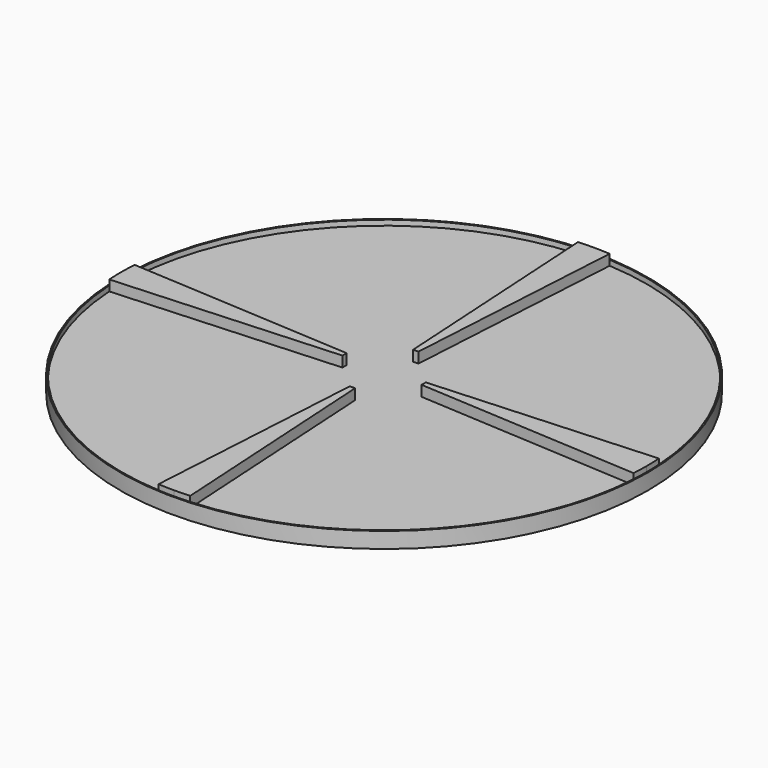
from build123d import *

# Parameters (mm, degrees)
F0_W      = 150
F0_H      = 140
F1_DEPTH  = 2
F2_R      = 2.5
F3_DEPTH  = 2.001
F4_R      = 50
F4_R_2    = 49.75
F5_DEPTH  = 1
F7_DEPTH  = 2
F8_DEPTH  = 25
F9_DEPTH  = 2.001
F10_DEPTH = 25


# Not quite as in the source:
# - a feature names something its author has since deleted; it is built from what else it names


with BuildPart() as f1:
    # F0 (on Top) → F1 (new body)
    with BuildSketch(Plane.XY):
        Rectangle(F0_W, F0_H)
    extrude(amount=F1_DEPTH)

    # F2 (on face) → F3 (cut, through all)
    with BuildSketch(Plane.XY.offset(2)):
        Polygon((-75, 70), (-75, 41.5), (-46.5, 70), align=None)
        with Locations((-64, 57.6)):
            Circle(F2_R, mode=Mode.SUBTRACT)
        Polygon((-46.5, -70), (-75, -41.5), (-75, -70), align=None)
        with Locations((-64, -57.6)):
            Circle(F2_R, mode=Mode.SUBTRACT)
        with BuildLine():
            Line((-67.1845650673, -7), (-67.1845650673, 7))
            ThreePointArc((-67.1845650673, 7), (-67.9167981143, 8.767766953), (-69.6845650673, 9.5))
            Line((-69.6845650673, 9.5), (-75, 9.5))
            Line((-75, 9.5), (-75, -9.5))
            Line((-75, -9.5), (-69.6845650673, -9.5))
            ThreePointArc((-69.6845650673, -9.5), (-67.9167981143, -8.767766953), (-67.1845650673, -7))
        make_face()
        with BuildLine():
            Line((-26.5348799016, -66.5942596452), (-27.945, -70))
            Line((-27.945, -70), (-15, -70))
            Line((-15, -70), (-16.5005719841, -66.5208040123))
            ThreePointArc((-16.5005719841, -66.5208040123), (-21.5420765789, -63.2311459437), (-26.5348799016, -66.5942596452))
        make_face()
        with BuildLine():
            Line((-15, 70), (-27.945, 70))
            Line((-27.945, 70), (-26.6428877925, 66.4417666182))
            ThreePointArc((-26.6428877925, 66.4417666182), (-21.596779976, 63.2315774362), (-16.6462859149, 66.5873377421))
            Line((-16.6462859149, 66.5873377421), (-15, 70))
        make_face()
        with Locations((-64, 57.6)):
            Circle(F2_R)
        with Locations((-64, -57.6)):
            Circle(F2_R)
    extrude(amount=-F3_DEPTH, mode=Mode.SUBTRACT)

    # F4 (on face) → F5 (join)
    with BuildSketch(Plane.XY.offset(2)):
        with Locations((-3.16328, 0)):
            Circle(F4_R)
        with Locations((-3.16328, 0)):
            Circle(F4_R_2, mode=Mode.SUBTRACT)
    extrude(amount=F5_DEPTH)

    # F6 (on face) → F7 (join)
    with BuildSketch(Plane.XY.offset(2)):
        with BuildLine():
            Line((-3.16328, 49.75), (-3.16328, 7.5))
            Line((-3.16328, 7.5), (-2.66328, 7.5))
            Line((-2.66328, 7.5), (-0.16328, 49.6594653616))
            ThreePointArc((-0.16328, 49.6594653616), (-1.662597112, 49.7273611895), (-3.16328, 49.75))
        make_face()
        with BuildLine():
            Line((46.58672, 0), (4.33672, 0))
            Line((4.33672, 0), (4.33672, -0.5))
            Line((4.33672, -0.5), (46.4961853616, -3))
            ThreePointArc((46.4961853616, -3), (46.5640811895, -1.500682888), (46.58672, 0))
        make_face()
        with BuildLine():
            ThreePointArc((-52.8227453616, 3), (-52.8906411895, 1.500682888), (-52.91328, 0))
            Line((-52.91328, 0), (-10.66328, 0))
            Line((-10.66328, 0), (-10.66328, 0.5))
            Line((-10.66328, 0.5), (-52.8227453616, 3))
        make_face()
        with BuildLine():
            Line((-3.66328, -7.5), (-6.16328, -49.6594653616))
            ThreePointArc((-6.16328, -49.6594653616), (-4.663962888, -49.7273611895), (-3.16328, -49.75))
            Line((-3.16328, -49.75), (-3.16328, -7.5))
            Line((-3.16328, -7.5), (-3.66328, -7.5))
        make_face()
        with BuildLine():
            Line((4.33672, 0.5), (4.33672, 0))
            Line((4.33672, 0), (46.58672, 0))
            ThreePointArc((46.58672, 0), (46.5640811895, 1.500682888), (46.4961853616, 3))
            Line((46.4961853616, 3), (4.33672, 0.5))
        make_face()
        with BuildLine():
            Line((-10.66328, 0), (-52.91328, 0))
            ThreePointArc((-52.91328, 0), (-52.8906411895, -1.500682888), (-52.8227453616, -3))
            Line((-52.8227453616, -3), (-10.66328, -0.5))
            Line((-10.66328, -0.5), (-10.66328, 0))
        make_face()
        with BuildLine():
            Line((-2.66328, -7.5), (-3.16328, -7.5))
            Line((-3.16328, -7.5), (-3.16328, -49.75))
            ThreePointArc((-3.16328, -49.75), (-1.662597112, -49.7273611895), (-0.16328, -49.6594653616))
            Line((-0.16328, -49.6594653616), (-2.66328, -7.5))
        make_face()
        with BuildLine():
            ThreePointArc((-3.16328, 49.75), (-4.663962888, 49.7273611895), (-6.16328, 49.6594653616))
            Line((-6.16328, 49.6594653616), (-3.66328, 7.5))
            Line((-3.66328, 7.5), (-3.16328, 7.5))
            Line((-3.16328, 7.5), (-3.16328, 49.75))
        make_face()
    extrude(amount=F7_DEPTH)

    # F2 (on face) → F8 (cut)
    with BuildSketch(Plane.XY.offset(2)):
        with Locations((-64, 57.6)):
            Circle(F2_R)
        with Locations((-64, -57.6)):
            Circle(F2_R)
        with BuildLine():
            Line((-15, 70), (-27.945, 70))
            Line((-27.945, 70), (-26.6428877925, 66.4417666182))
            ThreePointArc((-26.6428877925, 66.4417666182), (-21.596779976, 63.2315774362), (-16.6462859149, 66.5873377421))
            Line((-16.6462859149, 66.5873377421), (-15, 70))
        make_face()
        with BuildLine():
            Line((-26.5348799016, -66.5942596452), (-27.945, -70))
            Line((-27.945, -70), (-15, -70))
            Line((-15, -70), (-16.5005719841, -66.5208040123))
            ThreePointArc((-16.5005719841, -66.5208040123), (-21.5420765789, -63.2311459437), (-26.5348799016, -66.5942596452))
        make_face()
    extrude(amount=-F8_DEPTH, mode=Mode.SUBTRACT)

    # F2 (on face) + F4 (on face) → F9 (cut, through all)
    with BuildSketch(Plane.XY.offset(2)):
        with Locations((-64, 57.6)):
            Circle(F2_R)
        with Locations((-64, -57.6)):
            Circle(F2_R)
        with BuildLine():
            Line((-15, 70), (-27.945, 70))
            Line((-27.945, 70), (-26.6428877925, 66.4417666182))
            ThreePointArc((-26.6428877925, 66.4417666182), (-21.596779976, 63.2315774362), (-16.6462859149, 66.5873377421))
            Line((-16.6462859149, 66.5873377421), (-15, 70))
        make_face()
    with BuildSketch(Plane.XY.offset(2)):
        with BuildLine():
            Line((-16.5005719841, -66.5208040123), (-15, -70))
            Line((-15, -70), (75, -70))
            Line((75, -70), (75, 70))
            Line((75, 70), (-15, 70))
            Line((-15, 70), (-16.6462859149, 66.5873377421))
            ThreePointArc((-16.6462859149, 66.5873377421), (-21.596779976, 63.2315774362), (-26.6428877925, 66.4417666182))
            Line((-26.6428877925, 66.4417666182), (-27.945, 70))
            Line((-27.945, 70), (-46.5, 70))
            Line((-46.5, 70), (-75, 41.5))
            Line((-75, 41.5), (-75, 9.5))
            Line((-75, 9.5), (-69.6845650673, 9.5))
            ThreePointArc((-69.6845650673, 9.5), (-67.9167981143, 8.767766953), (-67.1845650673, 7))
            Line((-67.1845650673, 7), (-67.1845650673, -7))
            ThreePointArc((-67.1845650673, -7), (-67.9167981143, -8.767766953), (-69.6845650673, -9.5))
            Line((-69.6845650673, -9.5), (-75, -9.5))
            Line((-75, -9.5), (-75, -41.5))
            Line((-75, -41.5), (-46.5, -70))
            Line((-46.5, -70), (-27.945, -70))
            Line((-27.945, -70), (-26.5348799016, -66.5942596452))
            ThreePointArc((-26.5348799016, -66.5942596452), (-21.5420765789, -63.2311459437), (-16.5005719841, -66.5208040123))
        make_face()
        with Locations((-3.16328, 0)):
            Circle(F4_R, mode=Mode.SUBTRACT)
    extrude(amount=-F9_DEPTH, mode=Mode.SUBTRACT)

    # F2 (on face) + F0 (on Top) → F10 (cut)
    with BuildSketch(Plane.XY.offset(2)):
        Polygon((-46.5, -70), (-75, -41.5), (-75, -70), align=None)
        with Locations((-64, -57.6)):
            Circle(F2_R, mode=Mode.SUBTRACT)
        Polygon((-75, 70), (-75, 41.5), (-46.5, 70), align=None)
        with Locations((-64, 57.6)):
            Circle(F2_R, mode=Mode.SUBTRACT)
        with BuildLine():
            Line((-67.1845650673, -7), (-67.1845650673, 7))
            ThreePointArc((-67.1845650673, 7), (-67.9167981143, 8.767766953), (-69.6845650673, 9.5))
            Line((-69.6845650673, 9.5), (-75, 9.5))
            Line((-75, 9.5), (-75, -9.5))
            Line((-75, -9.5), (-69.6845650673, -9.5))
            ThreePointArc((-69.6845650673, -9.5), (-67.9167981143, -8.767766953), (-67.1845650673, -7))
        make_face()
        with BuildLine():
            Line((-26.5348799016, -66.5942596452), (-27.945, -70))
            Line((-27.945, -70), (-15, -70))
            Line((-15, -70), (-16.5005719841, -66.5208040123))
            ThreePointArc((-16.5005719841, -66.5208040123), (-21.5420765789, -63.2311459437), (-26.5348799016, -66.5942596452))
        make_face()
        with BuildLine():
            Line((-15, 70), (-27.945, 70))
            Line((-27.945, 70), (-26.6428877925, 66.4417666182))
            ThreePointArc((-26.6428877925, 66.4417666182), (-21.596779976, 63.2315774362), (-16.6462859149, 66.5873377421))
            Line((-16.6462859149, 66.5873377421), (-15, 70))
        make_face()
    with BuildSketch(Plane.XY):
        Rectangle(F0_W, F0_H)
    extrude(amount=-F10_DEPTH, mode=Mode.SUBTRACT)


solid = f1.part
